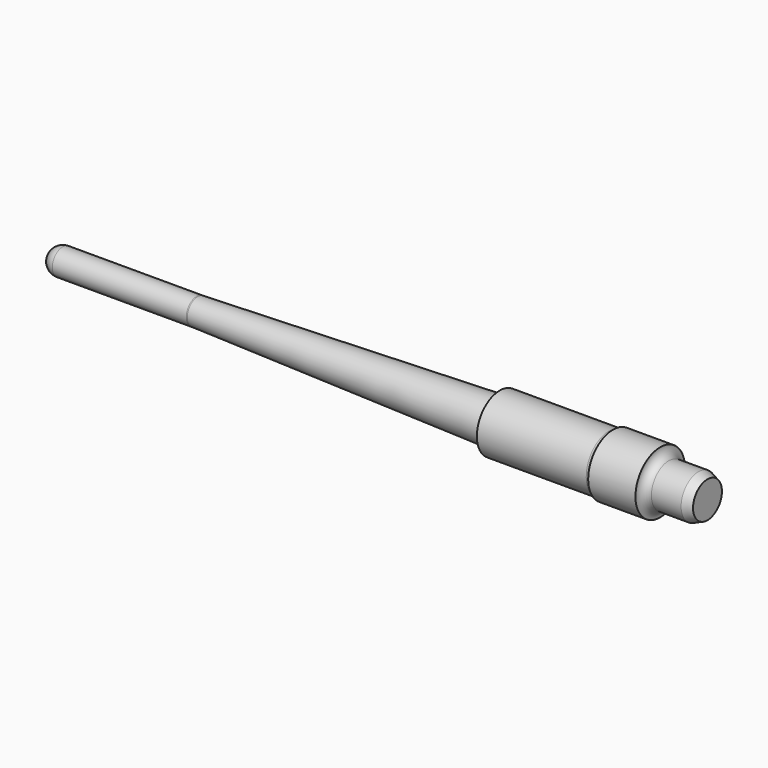
from build123d import *

# Parameters (mm, degrees)
F4_R     = 0.762
F5_SIZE2 = 0.3287820151
F5_SIZE  = 0.79375


# Not quite as in the source:
# - a fillet or chamfer that OpenCascade refuses, or shapes differently, is made with other operations: its cross-section is extruded or revolved along the edge and cut away or added


with BuildPart() as f1:
    # F0 (on Front) → F1 (revolve)
    with BuildSketch(Plane.XZ):
        with BuildLine():
            Line((-58.3184, 0), (0, 0))
            Line((0, 0), (0, 1.9304))
            Line((0, 1.9304), (-4.191, 1.9304))
            Line((-4.191, 1.9304), (-4.191, 2.7432))
            Line((-4.191, 2.7432), (-8.382, 2.7432))
            Line((-8.382, 2.7432), (-8.382, 2.54))
            Line((-8.382, 2.54), (-18.415, 2.54))
            Line((-18.415, 2.54), (-18.415, 1.9431))
            Line((-18.415, 1.9431), (-45.2374, 1.1557))
            Line((-45.2374, 1.1557), (-57.1627, 1.1557))
            ThreePointArc((-57.1627, 1.1557), (-57.979903307, 0.817203307), (-58.3184, 0))
        make_face()
    revolve(axis=Axis((-29.1592, 0, 0), (1, 0, 0)))

    # F2: fillet of radius 3.175 on 1 edges, made by hand

    # F2_s1 → F2_t2 (revolve)
    with BuildSketch(Plane.XZ):
        with BuildLine():
            ThreePointArc((-45.1908273531, 1.1570671894), (-45.2374050161, 1.1560418158), (-45.2839927102, 1.1557))
            Line((-45.2839927102, 1.1557), (-45.2374, 1.1557))
            Line((-45.2374, 1.1557), (-45.1908273531, 1.1570671894))
        make_face()
    revolve(axis=Axis((-45.2374, 0, 0), (1, 0, 0)))

    # F3: fillet of radius 0.381 on 2 edges, made by hand

    # F3_s1 → F3_t2 (revolve)
    with BuildSketch(Plane.XZ):
        with BuildLine():
            ThreePointArc((-18.7848201571, 1.9322435371), (-18.5226682235, 2.0476538916), (-18.415, 2.3130794743))
            Line((-18.415, 2.3130794743), (-18.40738, 2.3130794743))
            Line((-18.40738, 2.3130794743), (-18.40738, 1.9357004105))
            Line((-18.40738, 1.9357004105), (-18.7845965603, 1.9246268183))
            Line((-18.7845965603, 1.9246268183), (-18.7848201571, 1.9322435371))
        make_face()
    revolve(axis=Axis((-18.415, 0, 0), (1, 0, 0)))

    # F3_s3 → F3_t4 (revolve)
    with BuildSketch(Plane.XZ):
        with BuildLine():
            ThreePointArc((-8.7189690787, 2.54), (-8.5222215247, 2.5947310925), (-8.382, 2.7432))
            Line((-8.382, 2.7432), (-8.3752606184, 2.739644))
            ThreePointArc((-8.3752606184, 2.739644), (-8.37438, 2.6416), (-8.37438, 2.54))
            Line((-8.37438, 2.54), (-8.382, 2.53238))
            Line((-8.382, 2.53238), (-8.7189690787, 2.53238))
            Line((-8.7189690787, 2.53238), (-8.7189690787, 2.54))
        make_face()
    revolve(axis=Axis((-8.382, 0, 0), (1, 0, 0)))

    # F4
    f4_edges = [f1.edges().sort_by_distance(p)[0] for p in [
        (-4.191, 0, -1.9304),
    ]]
    fillet(f4_edges, radius=F4_R)

    # F5
    f5_edges = [f1.edges().sort_by_distance(p)[0] for p in [
        (0, 0, -1.9304),
    ]]
    chamfer(f5_edges, length=F5_SIZE, length2=F5_SIZE2)


solid = f1.part
